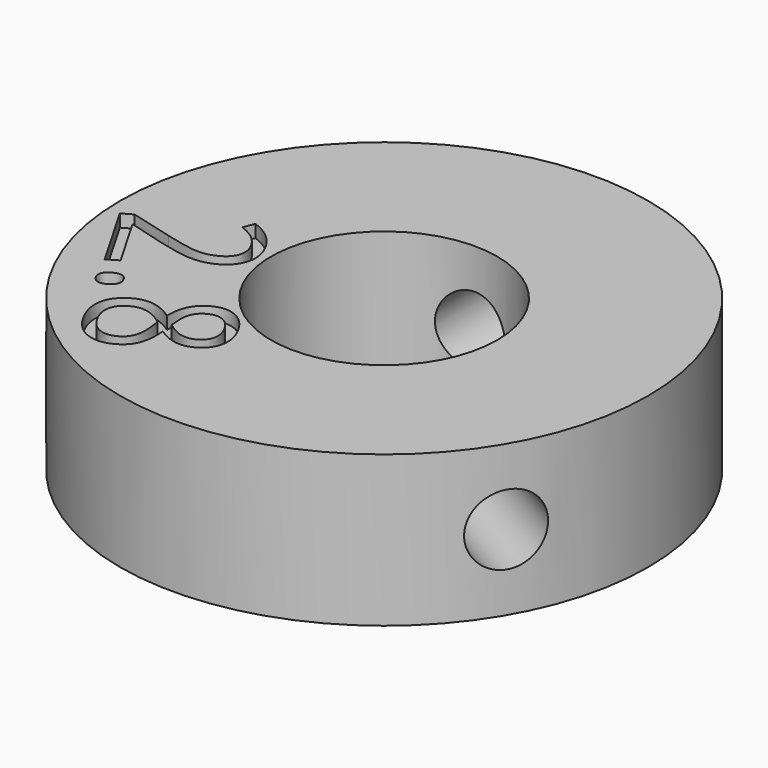
from build123d import *

# Parameters (mm, degrees)
F0_R          = 10.5
F0_R_2        = 4.5
F1_DEPTH      = 6
F7_R          = 1.4
F10_DEPTH     = 7.2233191439
F8_R          = 1.4
F11_DEPTH     = 7.2233191439
F9_R          = 1.4
F12_DEPTH     = 7.2233191439
F13_TEXT_SIZE = 6.6528012717
F14_DEPTH     = 0.5


# Not quite as in the source:
# - Text() gives the source's letters only with a copy of the font that has no kerning and outlines rounded to 1/6400 em; it was checked with that copy


with BuildPart() as f1:
    # F0 (on Top) → F1 (new body)
    with BuildSketch(Plane.XY):
        Circle(F0_R)
        Circle(F0_R_2, mode=Mode.SUBTRACT)
    extrude(amount=F1_DEPTH)

    # F7 (on line) → F10 (cut, up to face)
    with BuildSketch(Plane(origin=(9.0932667397, -5.25, 0), x_dir=(-0.5, -0.8660254038, 0), z_dir=(-0.8660254038, 0.5, 0))):
        with Locations((0, 3)):
            Circle(F7_R)
    extrude(amount=F10_DEPTH, mode=Mode.SUBTRACT)

    # F8 (on line) → F11 (cut, up to face)
    with BuildSketch(Plane(origin=(-9.0932667397, -5.25, 0), x_dir=(0.5, -0.8660254038, 0), z_dir=(-0.8660254038, -0.5, 0))):
        with Locations((0, 3)):
            Circle(F8_R)
    extrude(amount=-F11_DEPTH, mode=Mode.SUBTRACT)

    # F9 (on line) → F12 (cut, up to face)
    with BuildSketch(Plane(origin=(0, 10.5, 0), x_dir=(-1, 0, 0), z_dir=(0, 1, 0))):
        with Locations((0, 3)):
            Circle(F9_R)
    extrude(amount=-F12_DEPTH, mode=Mode.SUBTRACT)

    # F13 (on face) → F14 (cut)
    with BuildSketch(Plane.XY.offset(6)):
        with Locations(Location((-10.140337792, -0.3869595239), (0, 0, -60))):
            Text('2.8', F13_TEXT_SIZE, font='Open Sans', text_align=(TextAlign.LEFT, TextAlign.BOTTOM))
    extrude(amount=-F14_DEPTH, mode=Mode.SUBTRACT)


solid = f1.part
